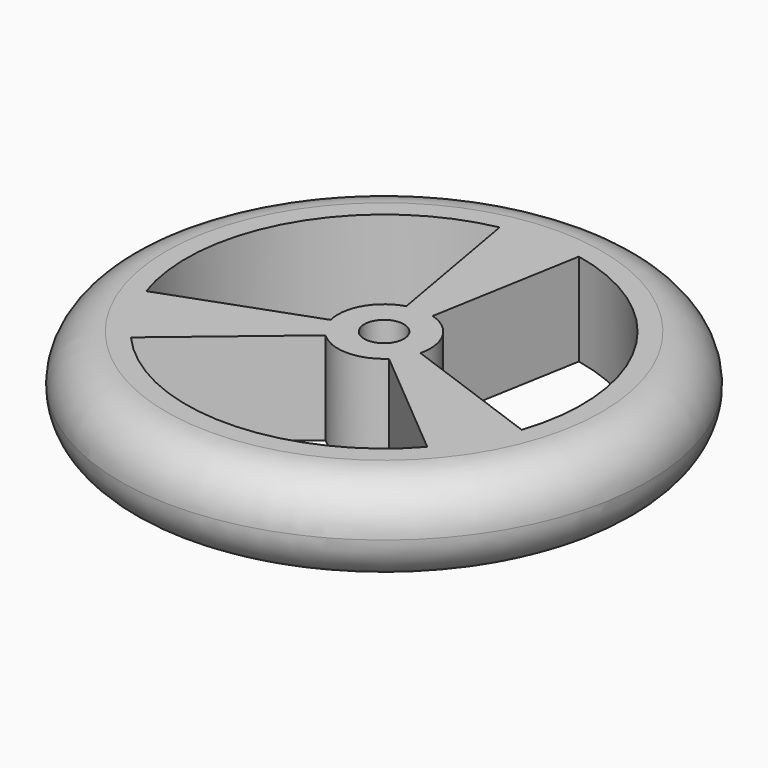
from build123d import *

# Parameters (mm, degrees)
F0_R     = 20
F0_R_2   = 1.5
F1_DEPTH = 7
F2_R     = 3.49999


# Not quite as in the source:
# - a fillet or chamfer is up to 0.001 mm smaller than in the source, because OpenCascade refuses the exact size


with BuildPart() as f1:
    # F0 (on Top) → F1 (new body)
    with BuildSketch(Plane.XY):
        Circle(F0_R)
        with BuildLine():
            Line((-11.2279220614, -9.9465454397), (-2.4047375097, -2.5430763869))
            ThreePointArc((-2.4047375097, -2.5430763869), (0, -3.5), (2.4047375097, -2.5430763869))
            Line((2.4047375097, -2.5430763869), (11.2279220614, -9.9465454397))
            ThreePointArc((11.2279220614, -9.9465454397), (0, -15), (-11.2279220614, -9.9465454397))
        make_face(mode=Mode.SUBTRACT)
        with BuildLine():
            ThreePointArc((-14.2279220614, -4.750393017), (-12.9903810568, 7.5), (-3, 14.6969384567))
            Line((-3, 14.6969384567), (-1, 3.3541019662))
            ThreePointArc((-1, 3.3541019662), (-3.0310889132, 1.75), (-3.4047375097, -0.8110255793))
            Line((-3.4047375097, -0.8110255793), (-14.2279220614, -4.750393017))
        make_face(mode=Mode.SUBTRACT)
        Circle(F0_R_2, mode=Mode.SUBTRACT)
        with BuildLine():
            ThreePointArc((3.4047375097, -0.8110255793), (3.0310889132, 1.75), (1, 3.3541019662))
            Line((1, 3.3541019662), (3, 14.6969384567))
            ThreePointArc((3, 14.6969384567), (12.9903810568, 7.5), (14.2279220614, -4.750393017))
            Line((14.2279220614, -4.750393017), (3.4047375097, -0.8110255793))
        make_face(mode=Mode.SUBTRACT)
    extrude(amount=F1_DEPTH)

    # F2 (radius 3.5 in the source; OpenCascade refuses exactly that, so slightly less here)
    f2_edges = [f1.edges().sort_by_distance(p)[0] for p in [
        (-20, 0, 7),
        (-20, 0, 0),
    ]]
    fillet(f2_edges, radius=F2_R)


solid = f1.part
